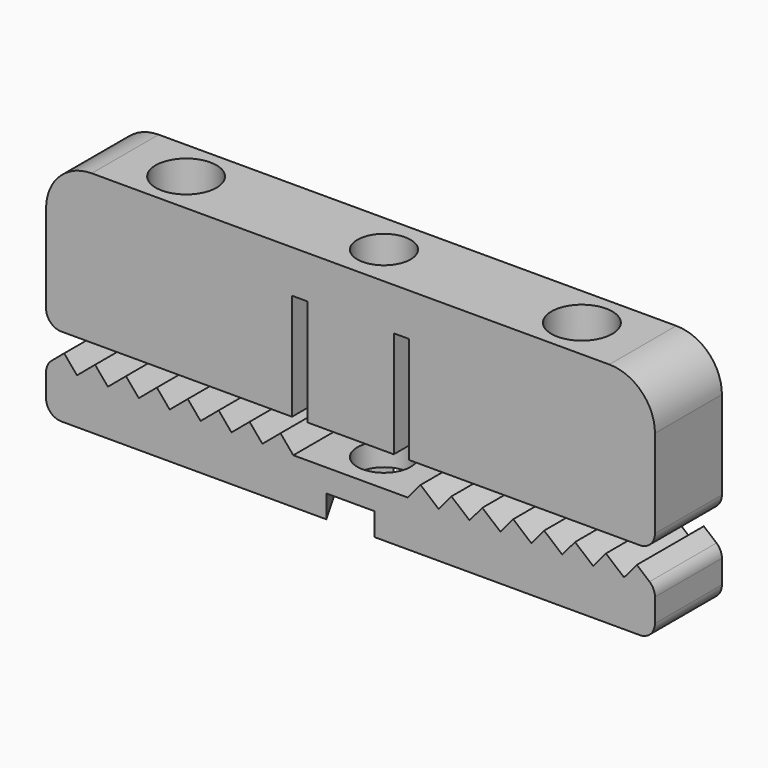
from build123d import *

# Parameters (mm, degrees)
F0_W      = 40
F0_H      = 5.5
F1_DEPTH  = 15
F3_DEPTH  = 6
F4_R      = 3
F5_R      = 2
F6_DEPTH  = 6
F7_R      = 1
F9_DEPTH  = 1.5
F10_R     = 1.75
F11_DEPTH = 25


# Not quite as in the source:
# - a feature names something its author has since deleted; it is built from what else it names


with BuildPart() as f1:
    # F0 (on Top) → F1 (new body)
    with BuildSketch(Plane.XY):
        Rectangle(F0_W, F0_H)
    extrude(amount=F1_DEPTH)

    # F2 (on face) → F3 (cut)
    with BuildSketch(Plane(origin=(0, 2.75, 0), x_dir=(-1, 0, 0), z_dir=(0, 1, 0))):
        Polygon((0, 3), (3.758946807, 3), (4.599775356, 4), (5.7890784562, 3), (6.6299070052, 4), (7.8192101053, 3), (8.6600386543, 4), (9.8493417544, 3), (10.6901703034, 4), (11.8794734035, 3), (12.7203019525, 4), (13.9096050526, 3), (14.7504336016, 4), (15.9397367018, 3), (16.7805652508, 4), (17.9698683509, 3), (18.8106968999, 4), (20, 3), (20, 5.2), (3.8406314086, 5.2), (3.8406314086, 12.2), (2.8406314086, 12.2), (2.8406314086, 5.2), (0, 5.2), (-2.8406314086, 5.2), (-2.8406314086, 12.2), (-3.8406314086, 12.2), (-3.8406314086, 5.2), (-20, 5.2), (-20, 3), (-18.8106968999, 4), (-17.9698683509, 3), (-16.7805652508, 4), (-15.9397367018, 3), (-14.7504336016, 4), (-13.9096050526, 3), (-12.7203019525, 4), (-11.8794734035, 3), (-10.6901703034, 4), (-9.8493417544, 3), (-8.6600386543, 4), (-7.8192101053, 3), (-6.6299070052, 4), (-5.7890784562, 3), (-4.599775356, 4), (-3.758946807, 3), align=None)
    extrude(amount=-F3_DEPTH, mode=Mode.SUBTRACT)

    # F4
    f4_edges = [f1.edges().sort_by_distance(p)[0] for p in [
        (-20, 0, 15),
        (20, 0, 15),
    ]]
    fillet(f4_edges, radius=F4_R)

    # F5 (on face) → F6 (cut)
    with BuildSketch(Plane.XY.offset(15)):
        with Locations((-13, 0)):
            Circle(F5_R)
        with Locations((13, 0)):
            Circle(F5_R)
    extrude(amount=-F6_DEPTH, mode=Mode.SUBTRACT)

    # F7
    f7_edges = [f1.edges().sort_by_distance(p)[0] for p in [
        (-20, 0, 5.2),
        (-20, 0, 0),
        (20, 0, 0),
        (20, 0, 5.2),
        (-20, 0, 3),
        (20, 0, 3),
    ]]
    fillet(f7_edges, radius=F7_R)

    # F8 (on face) → F9 (cut)
    with BuildSketch(Plane(origin=(0, 0, 0), x_dir=(1, 0, 0), z_dir=(0, 0, -1))):
        Polygon((-1.5877132403, -2.75), (1.5877132403, -2.75), (3.1754264805, 0), (1.5877132403, 2.75), (-1.5877132403, 2.75), (-3.1754264805, 0), align=None)
    extrude(amount=-F9_DEPTH, mode=Mode.SUBTRACT)

    # F10 (on face) → F11 (cut)
    with BuildSketch(Plane.XY.offset(15)):
        Circle(F10_R)
    extrude(amount=-F11_DEPTH, mode=Mode.SUBTRACT)


solid = f1.part
